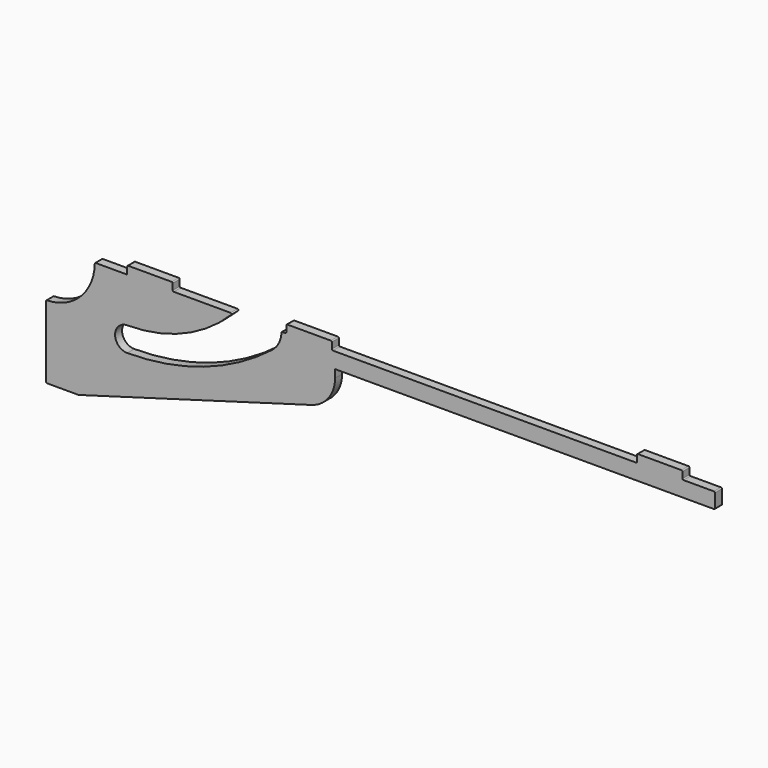
from build123d import *

# Parameters (mm, degrees)
F1_DEPTH = 3.429
F2_R     = 0.381


# Not quite as in the source:
# - ends of sketch curves that miss each other by under 0.0002 mm in the source are joined


with BuildPart() as f1:
    # F0 (on Front) → F1 (new body)
    with BuildSketch(Plane.XZ):
        with BuildLine():
            ThreePointArc((-523.3072592, 342.1259096), (-528.0697592, 346.8884096), (-523.3072592, 351.6509096))
            ThreePointArc((-523.3072592, 351.6509096), (-500.8987443088, 356.1961233076), (-482.0322439898, 369.1133948419))
            Line((-482.0322439898, 369.1133948419), (-505.5272592, 369.1134096))
            Line((-505.5272592, 369.1134096), (-505.5272592, 372.2884096))
            Line((-505.5272592, 372.2884096), (-523.3072592, 372.2884096))
            Line((-523.3072592, 372.2884096), (-523.3072592, 369.1134096))
            Line((-523.3072592, 369.1134096), (-536.0072592, 369.1134096))
            ThreePointArc((-536.0072592, 369.1134096), (-541.5868750184, 355.6430254184), (-555.0572592, 350.0634096))
            Line((-555.0572592, 350.0634096), (-555.0572592, 321.4884096))
            Line((-555.0572592, 321.4884096), (-542.3572592, 321.4884096))
            Line((-542.3572592, 321.4884096), (-451.219951, 347.675962))
            ThreePointArc((-451.219951, 347.675962), (-444.5824868492, 352.2417976203), (-442.0272592, 359.882059))
            Line((-442.0272592, 359.882059), (-442.0272592, 363.0174096))
            Line((-442.0272592, 363.0174096), (-293.4372592, 363.0174096))
            Line((-293.4372592, 363.0174096), (-293.4372592, 369.1134096))
            Line((-293.4372592, 369.1134096), (-306.1372592, 369.1134096))
            Line((-306.1372592, 369.1134096), (-306.1372592, 372.2884096))
            Line((-306.1372592, 372.2884096), (-323.9172592, 372.2884096))
            Line((-323.9172592, 372.2884096), (-323.9172592, 369.1134096))
            Line((-323.9172592, 369.1134096), (-443.2972592, 369.1134096))
            Line((-443.2972592, 369.1134096), (-443.2972592, 372.2884096))
            Line((-443.2972592, 372.2884096), (-461.0772592, 372.2884096))
            Line((-461.0772592, 372.2884096), (-461.0772592, 369.1134096))
            Line((-461.0772592, 369.1134096), (-462.9822592, 369.1134096))
            ThreePointArc((-462.9822592, 369.1134096), (-463.9484088233, 364.9334927075), (-466.650858723, 361.601539097))
            ThreePointArc((-466.650858723, 361.601539097), (-493.3520932085, 347.1307312076), (-523.3072592, 342.1259096))
        make_face()
    extrude(amount=F1_DEPTH)

    # F2
    f2_edges = [f1.edges().sort_by_distance(p)[0] for p in [
        (-482.032244, -1.7145, 369.113395),
        (-461.077259, -1.7145, 372.28841),
        (-461.077259, -1.7145, 369.11341),
        (-462.982259, -1.7145, 369.11341),
        (-505.527259, -1.7145, 372.28841),
        (-523.307259, -1.7145, 372.28841),
        (-523.307259, -1.7145, 369.11341),
        (-536.007259, -1.7145, 369.11341),
        (-505.527259, -1.7145, 369.11341),
        (-555.057259, -1.7145, 350.06341),
        (-443.297259, -1.7145, 369.11341),
        (-443.297259, -1.7145, 372.28841),
        (-323.917259, -1.7145, 372.28841),
        (-306.137259, -1.7145, 372.28841),
        (-306.137259, -1.7145, 369.11341),
        (-323.917259, -1.7145, 369.11341),
        (-293.437259, -1.7145, 369.11341),
        (-293.437259, -1.7145, 363.01741),
        (-542.357259, -1.7145, 321.48841),
        (-555.057259, -1.7145, 321.48841),
    ]]
    fillet(f2_edges, radius=F2_R)


solid = f1.part
